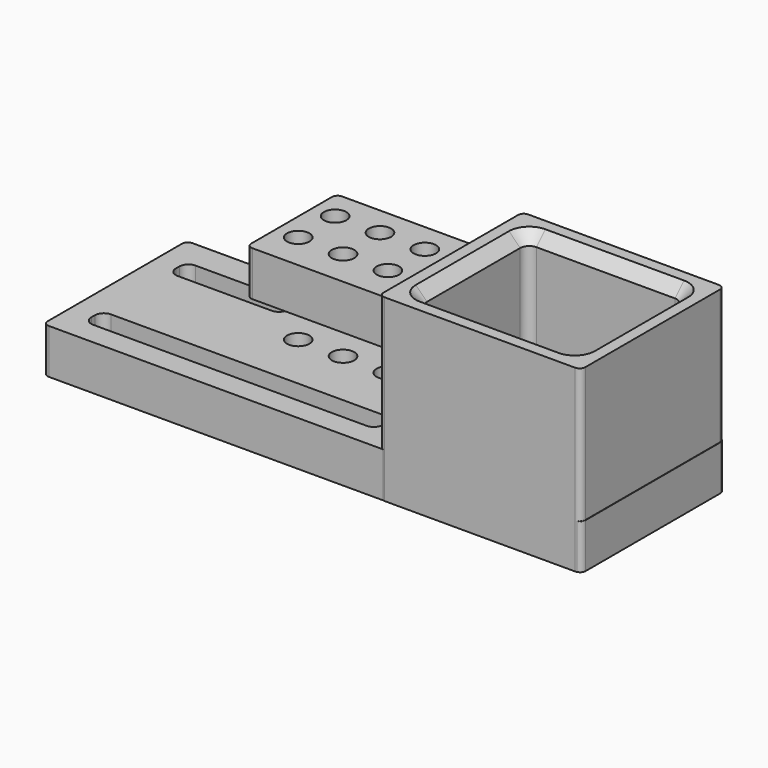
from build123d import *

# Parameters (mm, degrees)
F0_W          = 190.5
F0_H          = 101.6
F0_W_2        = 114.3
F0_W_3        = 88.9
F0_H_2        = 76.1922433317
F1_DEPTH      = 25.4
F2_W          = 114.3
F2_H          = 101.6530208289
F2_W_2        = 88.7144011029
F2_H_2        = 76.1204539018
F3_DEPTH      = 101.6
F4_W          = 63.5
F4_H          = 25.4
F5_DEPTH      = 126.4877107566
F6_W          = 21.1436580867
F6_H          = 30.0582610071
F7_DEPTH      = 108.712
F9_W          = 63.5019093752
F9_H          = 12.7
F9_W_2        = 165.1
F10_DEPTH     = 19.05
F12_R         = 6.35
F13_DEPTH     = 70.612
F14_T1_DEPTH  = 41.275
F14_T3_DEPTH  = 41.275
F14_T5_DEPTH  = 84.1375
F14_T10_DEPTH = 117.475
F14_T16_DEPTH = 117.475
F14_T22_DEPTH = 117.475
F14_T28_DEPTH = 84.1375
F14_T34_DEPTH = 84.1375
F14_T40_DEPTH = 84.1375
F14_T47_DEPTH = 84.1375
F14_T53_DEPTH = 84.1375
F14_T59_DEPTH = 117.475
F14_T65_DEPTH = 117.475
F14_T71_DEPTH = 117.475
F15_T1_DEPTH  = 40.8587766312
F15_T3_DEPTH  = 41.275
F16_R         = 5.08
F17_SIZE      = 6.35


# Not quite as in the source:
# - a fillet or chamfer that OpenCascade refuses, or shapes differently, is made with other operations: its cross-section is extruded or revolved along the edge and cut away or added


with BuildPart() as f1:
    # F0 (on Top) → F1 (new body)
    with BuildSketch(Plane.XY):
        with Locations((31.4233096536, -7.8402895808)):
            Rectangle(F0_W, F0_H)
        with Locations((183.8233096536, -7.8402895808)):
            Rectangle(F0_W_2, F0_H)
        with Locations((183.8233096536, -7.844167915)):
            Rectangle(F0_W_3, F0_H_2, mode=Mode.SUBTRACT)
        with Locations((183.8233096536, -7.844167915)):
            Rectangle(F0_W_3, F0_H_2)
    extrude(amount=F1_DEPTH)

    # F2 (on Top) → F3 (join)
    with BuildSketch(Plane.XY):
        with Locations((183.6377107566, -7.9463460934)):
            Rectangle(F2_W, F2_H)
        with Locations((183.7305102051, -7.8800626299)):
            Rectangle(F2_W_2, F2_H_2, mode=Mode.SUBTRACT)
    extrude(amount=F3_DEPTH)

    # F4 (on Right) → F5 (join, through all)
    with BuildSketch(Plane.YZ):
        with Locations((11.0370218754, 63.6608382941)):
            Rectangle(F4_W, F4_H)
    extrude(amount=F5_DEPTH)

    # F6 (on Front) → F7 (cut, symmetric)
    with BuildSketch(Plane.XZ):
        with Locations((10.5718290433, 63.3043590933)):
            Rectangle(F6_W, F6_H)
    extrude(amount=F7_DEPTH, both=True, mode=Mode.SUBTRACT)

    # F9 (on offset) → F10 (cut)
    with BuildSketch(Plane.XY.offset(25.4)):
        with Locations((-19.3757356588, 20.6727156579)):
            Rectangle(F9_W, F9_H)
        with Locations((31.4233096536, -39.1875091776)):
            Rectangle(F9_W_2, F9_H)
    extrude(amount=-F10_DEPTH, mode=Mode.SUBTRACT)

    # F12 (on offset) → F13 (cut)
    with BuildSketch(Plane.XY.offset(78.74)):
        with Locations((33.7039453115, 26.1378572217)):
            Circle(F12_R)
        with Locations((59.1039453115, 26.1378572217)):
            Circle(F12_R)
        with Locations((84.5039453115, 26.1378572217)):
            Circle(F12_R)
        with Locations((109.9039453115, 26.1378572217)):
            Circle(F12_R)
        with Locations((109.9039453115, 0)):
            Circle(F12_R)
        with Locations((84.5039453115, 0)):
            Circle(F12_R)
        with Locations((59.1039453115, 0)):
            Circle(F12_R)
        with Locations((33.7039453115, 0)):
            Circle(F12_R)
    extrude(amount=-F13_DEPTH, mode=Mode.SUBTRACT)

    # F14: fillet of radius 3.175 on 7 edges, made by hand

    # F14_s2 → F14_t1 (cut)
    with BuildSketch(Plane.XY.offset(43.0233382941)):
        with BuildLine():
            ThreePointArc((24.3186580867, -20.7129781246), (22.0735940564, -19.7830421549), (21.1436580867, -17.5379781246))
            Line((21.1436580867, -17.5379781246), (21.1436580867, -20.7129781246))
            Line((21.1436580867, -20.7129781246), (24.3186580867, -20.7129781246))
        make_face()
        with BuildLine():
            ThreePointArc((24.3186580867, 42.7870218754), (22.0735940564, 41.8570859056), (21.1436580867, 39.6120218754))
            Line((21.1436580867, 39.6120218754), (21.1436580867, 42.7870218754))
            Line((21.1436580867, 42.7870218754), (24.3186580867, 42.7870218754))
        make_face()
    extrude(amount=F14_T1_DEPTH, mode=Mode.SUBTRACT)

    # F14_s4 → F14_t3 (cut)
    with BuildSketch(Plane.XY.offset(-7.9375)):
        with BuildLine():
            ThreePointArc((240.9733096536, 39.7847104192), (240.0433736839, 42.0297744494), (237.7983096536, 42.9597104192))
            Line((237.7983096536, 42.9597104192), (240.9733096536, 42.9597104192))
            Line((240.9733096536, 42.9597104192), (240.9733096536, 39.7847104192))
        make_face()
    extrude(amount=F14_T3_DEPTH, mode=Mode.SUBTRACT)

    # F14_s6 → F14_t5 (cut)
    with BuildSketch(Plane.XY.offset(25.4)):
        with BuildLine():
            ThreePointArc((240.7877107566, 39.705164321), (239.8577747868, 41.9502283513), (237.6127107566, 42.880164321))
            Line((237.6127107566, 42.880164321), (240.7877107566, 42.880164321))
            Line((240.7877107566, 42.880164321), (240.7877107566, 39.705164321))
        make_face()
    extrude(amount=F14_T5_DEPTH, mode=Mode.SUBTRACT)


with BuildPart() as f14_tool8:
    # F14_s9 → F14_t10 (new body)
    with BuildSketch(Plane.XY.offset(-7.9375)):
        with BuildLine():
            ThreePointArc((126.4877107566, -55.5978565079), (127.4176467263, -57.8429205382), (129.6627107566, -58.7728565079))
            Line((129.6627107566, -58.7728565079), (126.4877107566, -58.7728565079))
            Line((126.4877107566, -58.7728565079), (126.4877107566, -55.5978565079))
        make_face()
    extrude(amount=F14_T10_DEPTH)

    split(bisect_by=Plane.XZ.offset(58.6402895808), keep=Keep.TOP)

    split(bisect_by=Plane.XY.offset(25.4), keep=Keep.BOTTOM)


with BuildPart() as f1_1:
    add(f1.part)

    # F14_t7: cut F14_tool8
    add(f14_tool8.part, mode=Mode.SUBTRACT)


with BuildPart() as f14_tool14:
    # F14_s15 → F14_t16 (new body)
    with BuildSketch(Plane.XY.offset(-7.9375)):
        with BuildLine():
            ThreePointArc((126.4877107566, -55.5978565079), (127.4176467263, -57.8429205382), (129.6627107566, -58.7728565079))
            Line((129.6627107566, -58.7728565079), (126.4877107566, -58.7728565079))
            Line((126.4877107566, -58.7728565079), (126.4877107566, -55.5978565079))
        make_face()
    extrude(amount=F14_T16_DEPTH)

    split(bisect_by=Plane.XZ.offset(58.6402895808), keep=Keep.BOTTOM)

    split(bisect_by=Plane.XY.offset(25.4), keep=Keep.TOP)


with BuildPart() as f1_2:
    add(f1_1.part)

    # F14_t13: cut F14_tool14
    add(f14_tool14.part, mode=Mode.SUBTRACT)


with BuildPart() as f14_tool20:
    # F14_s21 → F14_t22 (new body)
    with BuildSketch(Plane.XY.offset(-7.9375)):
        with BuildLine():
            ThreePointArc((126.4877107566, -55.5978565079), (127.4176467263, -57.8429205382), (129.6627107566, -58.7728565079))
            Line((129.6627107566, -58.7728565079), (126.4877107566, -58.7728565079))
            Line((126.4877107566, -58.7728565079), (126.4877107566, -55.5978565079))
        make_face()
    extrude(amount=F14_T22_DEPTH)

    split(bisect_by=Plane.XZ.offset(58.6402895808), keep=Keep.TOP)

    split(bisect_by=Plane.XY.offset(25.4), keep=Keep.TOP)


with BuildPart() as f1_3:
    add(f1_2.part)

    # F14_t19: cut F14_tool20
    add(f14_tool20.part, mode=Mode.SUBTRACT)


with BuildPart() as f14_tool26:
    # F14_s27 → F14_t28 (new body)
    with BuildSketch(Plane.XY.offset(25.4)):
        with BuildLine():
            ThreePointArc((126.4877107566, 39.705164321), (127.4176467263, 41.9502283513), (129.6627107566, 42.880164321))
            Line((129.6627107566, 42.880164321), (126.4877107566, 42.880164321))
            Line((126.4877107566, 42.880164321), (126.4877107566, 39.705164321))
        make_face()
    extrude(amount=F14_T28_DEPTH)

    split(bisect_by=Plane.XY.offset(50.9608382941), keep=Keep.BOTTOM)

    split(bisect_by=Plane.XZ.offset(-42.7870218754), keep=Keep.TOP)


with BuildPart() as f1_4:
    add(f1_3.part)

    # F14_t25: cut F14_tool26
    add(f14_tool26.part, mode=Mode.SUBTRACT)


with BuildPart() as f14_tool32:
    # F14_s33 → F14_t34 (new body)
    with BuildSketch(Plane.XY.offset(25.4)):
        with BuildLine():
            ThreePointArc((126.4877107566, 39.705164321), (127.4176467263, 41.9502283513), (129.6627107566, 42.880164321))
            Line((129.6627107566, 42.880164321), (126.4877107566, 42.880164321))
            Line((126.4877107566, 42.880164321), (126.4877107566, 39.705164321))
        make_face()
    extrude(amount=F14_T34_DEPTH)

    split(bisect_by=Plane.XY.offset(50.9608382941), keep=Keep.BOTTOM)

    split(bisect_by=Plane.XZ.offset(-42.7870218754), keep=Keep.BOTTOM)


with BuildPart() as f1_5:
    add(f1_4.part)

    # F14_t31: cut F14_tool32
    add(f14_tool32.part, mode=Mode.SUBTRACT)


with BuildPart() as f14_tool38:
    # F14_s39 → F14_t40 (new body)
    with BuildSketch(Plane.XY.offset(25.4)):
        with BuildLine():
            ThreePointArc((126.4877107566, 39.705164321), (127.4176467263, 41.9502283513), (129.6627107566, 42.880164321))
            Line((129.6627107566, 42.880164321), (126.4877107566, 42.880164321))
            Line((126.4877107566, 42.880164321), (126.4877107566, 39.705164321))
        make_face()
    extrude(amount=F14_T40_DEPTH)

    split(bisect_by=Plane.XY.offset(50.9608382941), keep=Keep.TOP)

    split(bisect_by=Plane.XZ.offset(-42.7870218754), keep=Keep.BOTTOM)

    split(bisect_by=Plane.XY.offset(76.3608382941), keep=Keep.BOTTOM)


with BuildPart() as f1_6:
    add(f1_5.part)

    # F14_t37: cut F14_tool38
    add(f14_tool38.part, mode=Mode.SUBTRACT)


with BuildPart() as f14_tool45:
    # F14_s46 → F14_t47 (new body)
    with BuildSketch(Plane.XY.offset(25.4)):
        with BuildLine():
            ThreePointArc((126.4877107566, 39.705164321), (127.4176467263, 41.9502283513), (129.6627107566, 42.880164321))
            Line((129.6627107566, 42.880164321), (126.4877107566, 42.880164321))
            Line((126.4877107566, 42.880164321), (126.4877107566, 39.705164321))
        make_face()
    extrude(amount=F14_T47_DEPTH)

    split(bisect_by=Plane.XZ.offset(-42.7870218754), keep=Keep.TOP)

    split(bisect_by=Plane.XY.offset(76.3608382941), keep=Keep.TOP)


with BuildPart() as f1_7:
    add(f1_6.part)

    # F14_t44: cut F14_tool45
    add(f14_tool45.part, mode=Mode.SUBTRACT)


with BuildPart() as f14_tool51:
    # F14_s52 → F14_t53 (new body)
    with BuildSketch(Plane.XY.offset(25.4)):
        with BuildLine():
            ThreePointArc((126.4877107566, 39.705164321), (127.4176467263, 41.9502283513), (129.6627107566, 42.880164321))
            Line((129.6627107566, 42.880164321), (126.4877107566, 42.880164321))
            Line((126.4877107566, 42.880164321), (126.4877107566, 39.705164321))
        make_face()
    extrude(amount=F14_T53_DEPTH)

    split(bisect_by=Plane.XZ.offset(-42.7870218754), keep=Keep.BOTTOM)

    split(bisect_by=Plane.XY.offset(76.3608382941), keep=Keep.TOP)


with BuildPart() as f1_8:
    add(f1_7.part)

    # F14_t50: cut F14_tool51
    add(f14_tool51.part, mode=Mode.SUBTRACT)


with BuildPart() as f14_tool57:
    # F14_s58 → F14_t59 (new body)
    with BuildSketch(Plane.XY.offset(-7.9375)):
        with BuildLine():
            ThreePointArc((237.6127107566, -58.7728565079), (239.8577747868, -57.8429205382), (240.7877107566, -55.5978565079))
            Line((240.7877107566, -55.5978565079), (240.7877107566, -58.7728565079))
            Line((240.7877107566, -58.7728565079), (237.6127107566, -58.7728565079))
        make_face()
    extrude(amount=F14_T59_DEPTH)

    split(bisect_by=Plane.XY.offset(25.4), keep=Keep.BOTTOM)

    split(bisect_by=Plane.XZ.offset(58.6402895808), keep=Keep.TOP)


with BuildPart() as f1_9:
    add(f1_8.part)

    # F14_t56: cut F14_tool57
    add(f14_tool57.part, mode=Mode.SUBTRACT)


with BuildPart() as f14_tool63:
    # F14_s64 → F14_t65 (new body)
    with BuildSketch(Plane.XY.offset(-7.9375)):
        with BuildLine():
            ThreePointArc((237.6127107566, -58.7728565079), (239.8577747868, -57.8429205382), (240.7877107566, -55.5978565079))
            Line((240.7877107566, -55.5978565079), (240.7877107566, -58.7728565079))
            Line((240.7877107566, -58.7728565079), (237.6127107566, -58.7728565079))
        make_face()
    extrude(amount=F14_T65_DEPTH)

    split(bisect_by=Plane.XY.offset(25.4), keep=Keep.TOP)

    split(bisect_by=Plane.XZ.offset(58.6402895808), keep=Keep.TOP)


with BuildPart() as f1_10:
    add(f1_9.part)

    # F14_t62: cut F14_tool63
    add(f14_tool63.part, mode=Mode.SUBTRACT)


with BuildPart() as f14_tool69:
    # F14_s70 → F14_t71 (new body)
    with BuildSketch(Plane.XY.offset(-7.9375)):
        with BuildLine():
            ThreePointArc((237.6127107566, -58.7728565079), (239.8577747868, -57.8429205382), (240.7877107566, -55.5978565079))
            Line((240.7877107566, -55.5978565079), (240.7877107566, -58.7728565079))
            Line((240.7877107566, -58.7728565079), (237.6127107566, -58.7728565079))
        make_face()
    extrude(amount=F14_T71_DEPTH)

    split(bisect_by=Plane.XY.offset(25.4), keep=Keep.TOP)

    split(bisect_by=Plane.XZ.offset(58.6402895808), keep=Keep.BOTTOM)


with BuildPart() as f1_11:
    add(f1_10.part)

    # F14_t68: cut F14_tool69
    add(f14_tool69.part, mode=Mode.SUBTRACT)

    # F15: fillet of radius 3.175 on 3 edges, made by hand

    # F15_s2 → F15_t1 (cut)
    with BuildSketch(Plane.XY.offset(-7.7293883156)):
        with BuildLine():
            ThreePointArc((238.5205796881, -58.6402895808), (240.2856608913, -57.5217825462), (240.9733096536, -55.5485342546))
            Line((240.9733096536, -55.5485342546), (241.0368096536, -55.5485342546))
            Line((241.0368096536, -55.5485342546), (241.0368096536, -58.6402895808))
            Line((241.0368096536, -58.6402895808), (240.9733096536, -58.7037895808))
            ThreePointArc((240.9733096536, -58.7037895808), (239.7469446708, -58.7037895808), (238.5350250887, -58.7021246873))
            Line((238.5350250887, -58.7021246873), (238.5205796881, -58.6402895808))
        make_face()
    extrude(amount=F15_T1_DEPTH, mode=Mode.SUBTRACT)

    # F15_s4 → F15_t3 (cut)
    with BuildSketch(Plane.XY.offset(-7.9375)):
        with BuildLine():
            ThreePointArc((-60.6516903464, -58.6402895808), (-62.8967543766, -57.7103536111), (-63.8266903464, -55.4652895808))
            Line((-63.8266903464, -55.4652895808), (-63.8901903464, -55.4652895808))
            Line((-63.8901903464, -55.4652895808), (-63.8901903464, -58.7037895808))
            Line((-63.8901903464, -58.7037895808), (-60.6516903464, -58.7037895808))
            Line((-60.6516903464, -58.7037895808), (-60.6516903464, -58.6402895808))
        make_face()
        with BuildLine():
            ThreePointArc((-60.6516903464, 42.9597104192), (-62.8967543766, 42.0297744494), (-63.8266903464, 39.7847104192))
            Line((-63.8266903464, 39.7847104192), (-63.8901903464, 39.7847104192))
            Line((-63.8901903464, 39.7847104192), (-63.8901903464, 43.0232104192))
            Line((-63.8901903464, 43.0232104192), (-60.6516903464, 43.0232104192))
            Line((-60.6516903464, 43.0232104192), (-60.6516903464, 42.9597104192))
        make_face()
    extrude(amount=F15_T3_DEPTH, mode=Mode.SUBTRACT)

    # F16
    f16_edges = [f1_11.edges().sort_by_distance(p)[0] for p in [
        (12.375219, 27.022716, 15.875),
        (12.375219, 14.322716, 15.875),
        (-51.12669, 27.022716, 15.875),
        (-51.12669, 14.322716, 15.875),
        (-51.12669, -32.837509, 15.875),
        (-51.12669, -45.537509, 15.875),
        (113.97331, -32.837509, 15.875),
        (113.97331, -45.537509, 15.875),
        (126.487711, -20.712978, 63.660838),
        (139.37331, 30.180164, 63.5),
        (139.37331, -45.94029, 63.5),
        (228.087711, 30.180164, 63.5),
        (228.087711, -45.94029, 63.5),
    ]]
    fillet(f16_edges, radius=F16_R)

    # F17
    f17_edges = [f1_11.edges().sort_by_distance(p)[0] for p in [
        (139.37331, -7.880063, 101.6),
    ]]
    chamfer(f17_edges, length=F17_SIZE)


solid = f1_11.part
